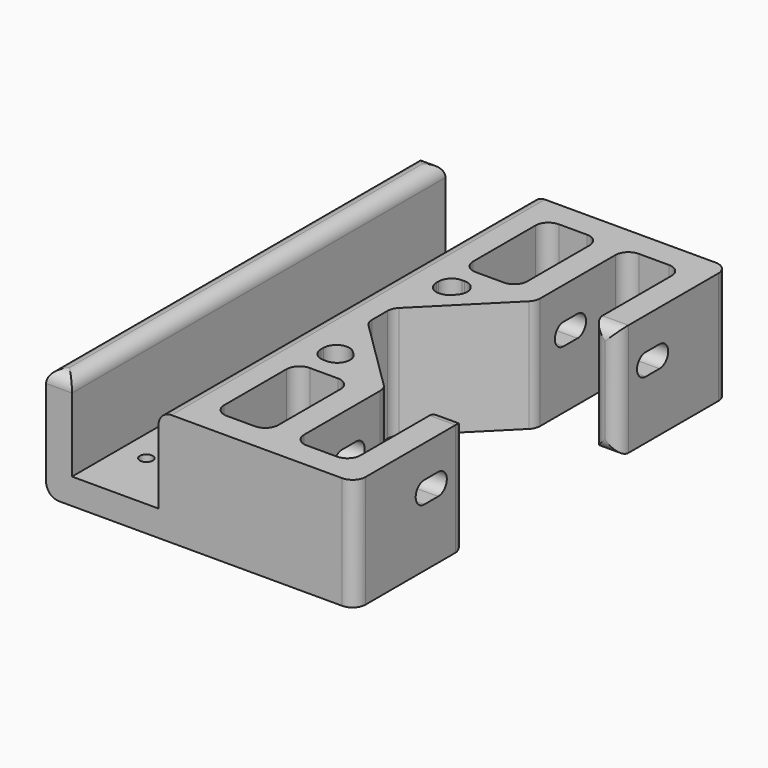
from build123d import *

# Parameters (mm, degrees)
F0_W     = 12.5
F0_H     = 24
F1_DEPTH = 6
F0_W_2   = 20
F0_H_2   = 108
F0_R     = 1.5
F0_W_3   = 6
F2_DEPTH = 26
F5_DEPTH = 30
F6_R     = 2.99999


# Not quite as in the source:
# - a fillet or chamfer is up to 0.001 mm smaller than in the source, because OpenCascade refuses the exact size


with BuildPart() as f1:
    # F0 (on Top) → F1 (new body)
    with BuildSketch(Plane.XY):
        with Locations((6.25, -36)):
            Rectangle(F0_W, F0_H)
    extrude(amount=F1_DEPTH)



with BuildPart() as f1b:
    # F0 (on Top) → F1, piece 2 (new body)
    with BuildSketch(Plane.XY):
        Polygon((11.0289425277, -20), (0, -9.1190332702), (0, -20), align=None)
    extrude(amount=F1_DEPTH)


with BuildPart() as f1c:
    # F0 (on Top) → F1, piece 3 (new body)
    with BuildSketch(Plane.XY):
        with Locations((6.25, 36)):
            Rectangle(F0_W, F0_H)
    extrude(amount=F1_DEPTH)


with BuildPart() as f1d:
    # F0 (on Top) → F1, piece 4 (new body)
    with BuildSketch(Plane.XY):
        with Locations((-18, 0)):
            Rectangle(F0_W_2, F0_H_2)
        with Locations((-22, -40)):
            Circle(F0_R, mode=Mode.SUBTRACT)
        with Locations((-14, -40)):
            Circle(F0_R, mode=Mode.SUBTRACT)
        with Locations((-22, -20)):
            Circle(F0_R, mode=Mode.SUBTRACT)
        with Locations((-14, -20)):
            Circle(F0_R, mode=Mode.SUBTRACT)
        with Locations((-22, 0)):
            Circle(F0_R, mode=Mode.SUBTRACT)
        with Locations((-22, 20)):
            Circle(F0_R, mode=Mode.SUBTRACT)
        with Locations((-14, 0)):
            Circle(F0_R, mode=Mode.SUBTRACT)
        with Locations((-14, 20)):
            Circle(F0_R, mode=Mode.SUBTRACT)
        with Locations((-22, 40)):
            Circle(F0_R, mode=Mode.SUBTRACT)
        with Locations((-14, 40)):
            Circle(F0_R, mode=Mode.SUBTRACT)
    extrude(amount=F1_DEPTH)


with BuildPart() as f1e:
    # F0 (on Top) → F1, piece 5 (new body)
    with BuildSketch(Plane.XY):
        Polygon((0, 20), (0, 9.1568542495), (10.8431457505, 20), align=None)
    extrude(amount=F1_DEPTH)


with BuildPart() as f1_1:
    add(f1.part)

    add(f1b.part)  # F2 merges F1b

    add(f1c.part)  # F2 merges F1c

    add(f1d.part)  # F2 merges F1d

    add(f1e.part)  # F2 merges F1e
    # F0 (on Top) → F2 (join)
    with BuildSketch(Plane.XY):
        Polygon((18.5, 22), (18.5, 48), (31.5, 48), (31.5, 22), (37.5, 22), (37.5, 54), (-8, 54), (-8, -54), (37.5, -54), (37.5, -22), (31.5, -22), (31.5, -48), (18.5, -48), (18.5, -21.7517847015), (0, -3.5), (0, 3.5), align=None)
        with Locations((6.25, -36)):
            Rectangle(F0_W, F0_H, mode=Mode.SUBTRACT)
        Polygon((0, -20), (0, -9.1190332702), (11.0289425277, -20), align=None, mode=Mode.SUBTRACT)
        Polygon((10.8431457505, 20), (0, 9.1568542495), (0, 20), align=None, mode=Mode.SUBTRACT)
        with Locations((6.25, 36)):
            Rectangle(F0_W, F0_H, mode=Mode.SUBTRACT)
        with Locations((-31, 0)):
            Rectangle(F0_W_3, F0_H_2)
    extrude(amount=F2_DEPTH)

    # F4 (on offset) → F5 (cut)
    with BuildSketch(Plane.YZ.offset(37.5)):
        with BuildLine():
            ThreePointArc((-34, 18.5), (-36.5, 16), (-34, 13.5))
            Line((-34, 13.5), (-30, 13.5))
            ThreePointArc((-30, 13.5), (-27.5, 16), (-30, 18.5))
            Line((-30, 18.5), (-34, 18.5))
        make_face()
        with BuildLine():
            Line((34, 18.5), (30, 18.5))
            ThreePointArc((30, 18.5), (27.5, 16), (30, 13.5))
            Line((30, 13.5), (34, 13.5))
            ThreePointArc((34, 13.5), (36.5, 16), (34, 18.5))
        make_face()
    extrude(amount=-F5_DEPTH, mode=Mode.SUBTRACT)

    # F6 (radius 3 in the source; OpenCascade refuses exactly that, so slightly less here)
    f6_edges = [f1_1.edges().sort_by_distance(p)[0] for p in [
        (0, 48, 16),
        (18.5, 48, 13),
        (31.5, 48, 13),
        (12.5, 48, 16),
        (12.5, -24, 16),
        (0, -24, 16),
        (0, 20, 16),
        (0, -9.119033, 16),
        (0, -20, 16),
        (11.028943, -20, 16),
        (10.843146, 20, 16),
        (0, 9.156854, 16),
        (0, -48, 16),
        (18.5, -48, 13),
        (0, 24, 16),
        (12.5, 24, 16),
        (12.5, -48, 16),
        (31.5, -48, 13),
        (37.5, -54, 13),
        (37.5, 54, 13),
        (34.5, 22, 26),
        (34.5, -22, 26),
        (34.5, -22, 0),
        (34.5, 22, 0),
        (0, -3.5, 13),
        (0, 3.5, 13),
        (18.5, -21.751785, 13),
        (18.5, 22, 13),
        (31.5, 22, 13),
        (37.5, 22, 13),
        (31.5, -22, 13),
        (37.5, -22, 13),
        (-31, -54, 26),
        (-31, 54, 26),
        (-34, 0, 0),
        (-28, 0, 26),
        (-8, 0, 26),
        (-34, 0, 26),
    ]]
    fillet(f6_edges, radius=F6_R)


solid = f1_1.part
